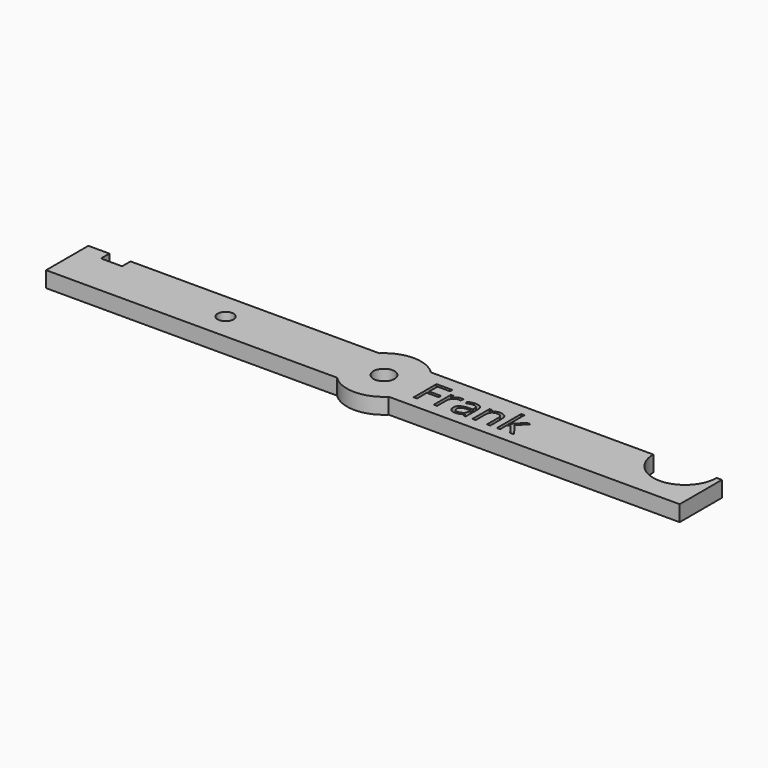
from build123d import *

# Parameters (mm, degrees)
F0_R         = 1.5
F0_R_2       = 2
F1_DEPTH     = 3
F2_TEXT_SIZE = 7.5701074416
F3_DEPTH     = 25


# Not quite as in the source:
# - Text() gives the source's letters only with a copy of the font that has no kerning and outlines rounded to 1/6400 em; it was checked with that copy


with BuildPart() as f1:
    # F0 (on Top) → F1 (new body)
    with BuildSketch(Plane.XY):
        with BuildLine():
            Line((-60, 5), (-60, -5))
            Line((-60, -5), (-4.8989794856, -5))
            ThreePointArc((-4.8989794856, -5), (-7, 0), (-4.8989794856, 5))
            Line((-4.8989794856, 5), (-52, 5))
            Line((-52, 5), (-52, 3))
            Line((-52, 3), (-56, 3))
            Line((-56, 3), (-56, 5))
            Line((-56, 5), (-60, 5))
        make_face()
        with Locations((-30, 0)):
            Circle(F0_R, mode=Mode.SUBTRACT)
        with BuildLine():
            ThreePointArc((7, 0), (6.4534043883, -2.7117470016), (4.8989794856, -5))
            Line((4.8989794856, -5), (60, -5))
            Line((60, -5), (60, 5))
            Line((60, 5), (59, 5))
            ThreePointArc((59, 5), (53, -1), (47, 5))
            Line((47, 5), (4.8989794856, 5))
            ThreePointArc((4.8989794856, 5), (6.4534043883, 2.7117470016), (7, 0))
        make_face()
        with BuildLine():
            Line((4.8989794856, -5), (-4.8989794856, -5))
            ThreePointArc((-4.8989794856, -5), (0, -7), (4.8989794856, -5))
        make_face()
        with BuildLine():
            ThreePointArc((-4.8989794856, 5), (-7, 0), (-4.8989794856, -5))
            Line((-4.8989794856, -5), (4.8989794856, -5))
            ThreePointArc((4.8989794856, -5), (6.4534043883, -2.7117470016), (7, 0))
            ThreePointArc((7, 0), (6.4534043883, 2.7117470016), (4.8989794856, 5))
            Line((4.8989794856, 5), (-4.8989794856, 5))
        make_face()
        Circle(F0_R_2, mode=Mode.SUBTRACT)
        with BuildLine():
            ThreePointArc((4.8989794856, 5), (0, 7), (-4.8989794856, 5))
            Line((-4.8989794856, 5), (4.8989794856, 5))
        make_face()
    extrude(amount=F1_DEPTH)

    # F2 (on face) → F3 (cut)
    with BuildSketch(Plane.XY.offset(3)):
        with Locations((7.1420059539, -2.8192123864)):
            Text('Frank', F2_TEXT_SIZE, font='Open Sans', text_align=(TextAlign.LEFT, TextAlign.BOTTOM))
    extrude(amount=-F3_DEPTH, mode=Mode.SUBTRACT)


solid = f1.part
